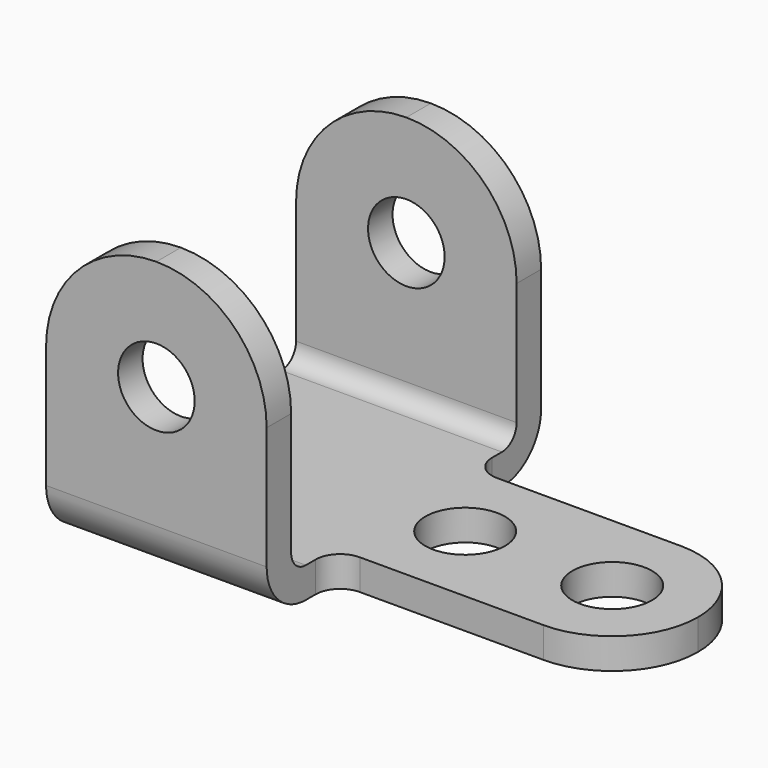
from build123d import *

# Parameters (mm, degrees)
F0_R     = 9.92251
F1_DEPTH = 44.45
F2_R     = 10.3251
F3_DEPTH = 7.9375
F4_W     = 73.025
F4_H     = 76.2
F5_DEPTH = 133.351
F6_R     = 12.7
F7_R     = 4.7625
F8_R     = 6.35


with BuildPart() as f1:
    # F0 (on Front) → F1 (new body, symmetric)
    with BuildSketch(Plane.XZ):
        with BuildLine():
            Line((0, 44.45), (0, 0))
            Line((0, 0), (57.15, 0))
            Line((57.15, 0), (57.15, 44.45))
            ThreePointArc((57.15, 44.45), (48.7805762724, 64.6555762724), (28.575, 73.025))
            ThreePointArc((28.575, 73.025), (8.3694237276, 64.6555762724), (0, 44.45))
        make_face()
        with Locations((28.575, 44.45)):
            Circle(F0_R, mode=Mode.SUBTRACT)
    extrude(amount=F1_DEPTH, both=True)

    # F2 (on Top) → F3 (join)
    with BuildSketch(Plane.XY):
        with BuildLine():
            Line((0, 22.225), (0, -22.225))
            Line((0, -22.225), (111.125, -22.225))
            ThreePointArc((111.125, -22.225), (126.8404482119, -15.7154482119), (133.35, 0))
            ThreePointArc((133.35, 0), (126.8404482119, 15.7154482119), (111.125, 22.225))
            Line((111.125, 22.225), (0, 22.225))
        make_face()
        with Locations((73.025, 0)):
            Circle(F2_R, mode=Mode.SUBTRACT)
        with Locations((111.125, 0)):
            Circle(F2_R, mode=Mode.SUBTRACT)
    extrude(amount=F3_DEPTH)

    # F4 (on Right) → F5 (cut, through all)
    with BuildSketch(Plane.YZ):
        with Locations((0, 46.0375)):
            Rectangle(F4_W, F4_H)
    extrude(amount=F5_DEPTH, mode=Mode.SUBTRACT)

    # F6
    f6_edges = [f1.edges().sort_by_distance(p)[0] for p in [
        (28.575, -44.45, 0),
        (28.575, 44.45, 0),
    ]]
    fillet(f6_edges, radius=F6_R)

    # F7
    f7_edges = [f1.edges().sort_by_distance(p)[0] for p in [
        (28.575, 36.5125, 7.9375),
        (28.575, -36.5125, 7.9375),
    ]]
    fillet(f7_edges, radius=F7_R)

    # F8
    f8_edges = [f1.edges().sort_by_distance(p)[0] for p in [
        (57.15, 22.225, 3.96875),
        (57.15, -22.225, 3.96875),
    ]]
    fillet(f8_edges, radius=F8_R)


solid = f1.part
